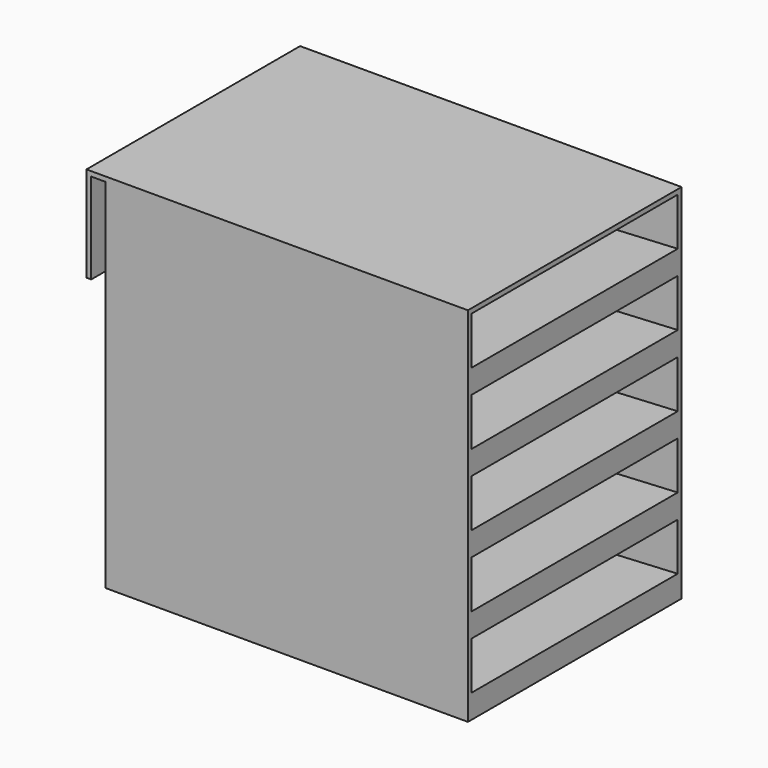
from build123d import *

# Parameters (mm, degrees)
F0_W           = 76
F0_H           = 76
F1_DEPTH       = 28
F2_W           = 54
F2_H           = 10
F5_W           = 56
F5_H           = 76
F6_DEPTH       = 1
F8_DEPTH       = 56
F9_TEXT_SIZE   = 8.9253324808
F9_TEXT_SIZE_2 = 9.2617753479
F9_TEXT_SIZE_3 = 9.3902593815
F9_TEXT_SIZE_4 = 9.6482923254
F9_TEXT_SIZE_5 = 10.8240379228
F10_DEPTH      = 1


# Not quite as in the source:
# - Text() gives the source's letters only with a copy of the font that has no kerning and outlines rounded to 1/6400 em; it was checked with that copy


with BuildPart() as f1:
    # F0 (on Front) → F1 (new body, symmetric)
    with BuildSketch(Plane.XZ):
        Rectangle(F0_W, F0_H)
    extrude(amount=F1_DEPTH, both=True)

    # F4: sweep along a path in F3
    with BuildLine(Plane.XZ.offset(28)) as f4_path:
        Line((38, 37), (-38, 33.0170087745))
    # F2 (on face) → F4 (sweep, cut)
    with BuildSketch(Plane.YZ.offset(38)):
        with Locations((0, 32)):
            Rectangle(F2_W, F2_H)
        with Locations((0, 17)):
            Rectangle(F2_W, F2_H)
        with Locations((0, 2)):
            Rectangle(F2_W, F2_H)
        with Locations((0, -13)):
            Rectangle(F2_W, F2_H)
        with Locations((0, -28)):
            Rectangle(F2_W, F2_H)
    sweep(path=f4_path.line, mode=Mode.SUBTRACT)

    # F5 (on face) → F6 (join)
    with BuildSketch(Plane(origin=(-38, 0, 0), x_dir=(0, -1, 0), z_dir=(-1, 0, 0))):
        Rectangle(F5_W, F5_H)
    extrude(amount=-F6_DEPTH)

    # F7 (on face) → F8 (join)
    with BuildSketch(Plane.XZ.offset(28)):
        Polygon((-38, 37), (-38, 38), (-42, 38), (-42, 18), (-41, 18), (-41, 37), align=None)
    extrude(amount=-F8_DEPTH)

    # F9 (on face) → F10 (join)
    with BuildSketch(Plane(origin=(0, 28, 0), x_dir=(-1, 0, 0), z_dir=(0, 1, 0))):
        with Locations((-30.6668113917, 28.5186786205)):
            Text('F', F9_TEXT_SIZE, font='Open Sans', text_align=(TextAlign.LEFT, TextAlign.BOTTOM))
        with Locations((-30.4371416569, 12.921391055)):
            Text('G', F9_TEXT_SIZE_2, font='Open Sans', text_align=(TextAlign.LEFT, TextAlign.BOTTOM))
        with Locations((-29.9739278853, -1.6359465662)):
            Text('H', F9_TEXT_SIZE_3, font='Open Sans', text_align=(TextAlign.LEFT, TextAlign.BOTTOM))
        with Locations((-29.9739278853, -16.6555196047)):
            Text('I/J', F9_TEXT_SIZE_4, font='Open Sans', text_align=(TextAlign.LEFT, TextAlign.BOTTOM))
        with Locations((-29.9739278853, -33.0321379006)):
            Text('K/L', F9_TEXT_SIZE_5, font='Open Sans', text_align=(TextAlign.LEFT, TextAlign.BOTTOM))
    extrude(amount=F10_DEPTH)


solid = f1.part
